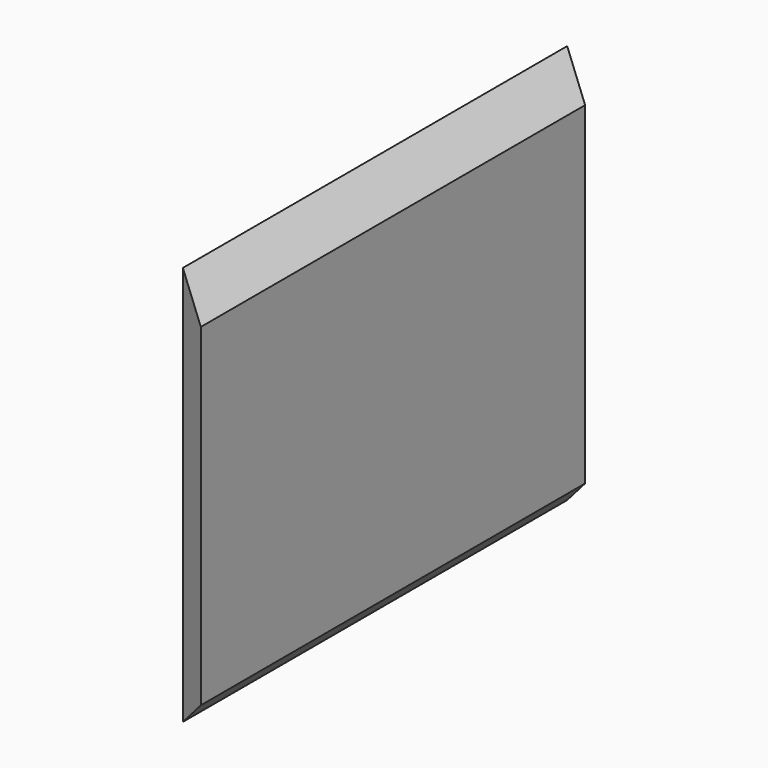
from build123d import *

# Parameters (mm, degrees)
F0_W     = 285.75
F0_H     = 228.6
F1_DEPTH = 19.05
F3_DEPTH = 228.601
F4_SIZE  = 19.04999


# Not quite as in the source:
# - a fillet or chamfer is up to 0.001 mm smaller than in the source, because OpenCascade refuses the exact size


with BuildPart() as f1:
    # F0 (on Right) → F1 (new body)
    with BuildSketch(Plane.YZ):
        Rectangle(F0_W, F0_H)
    extrude(amount=F1_DEPTH)

    # F2 (on face) → F3 (cut, through all)
    with BuildSketch(Plane.XY.offset(114.3)):
        Polygon((0, -142.875), (19.05, -142.875), (0, -131.8764773719), align=None)
        Polygon((19.05, 142.875), (0, 142.875), (19.05, 131.8764773719), align=None)
    extrude(amount=-F3_DEPTH, mode=Mode.SUBTRACT)

    # F4 (size 19.05 in the source; OpenCascade refuses exactly that, so slightly less here)
    f4_edges = [f1.edges().sort_by_distance(p)[0] for p in [
        (19.05, -5.499261, 114.3),
        (19.05, -5.499261, -114.3),
    ]]
    chamfer(f4_edges, length=F4_SIZE)


solid = f1.part
